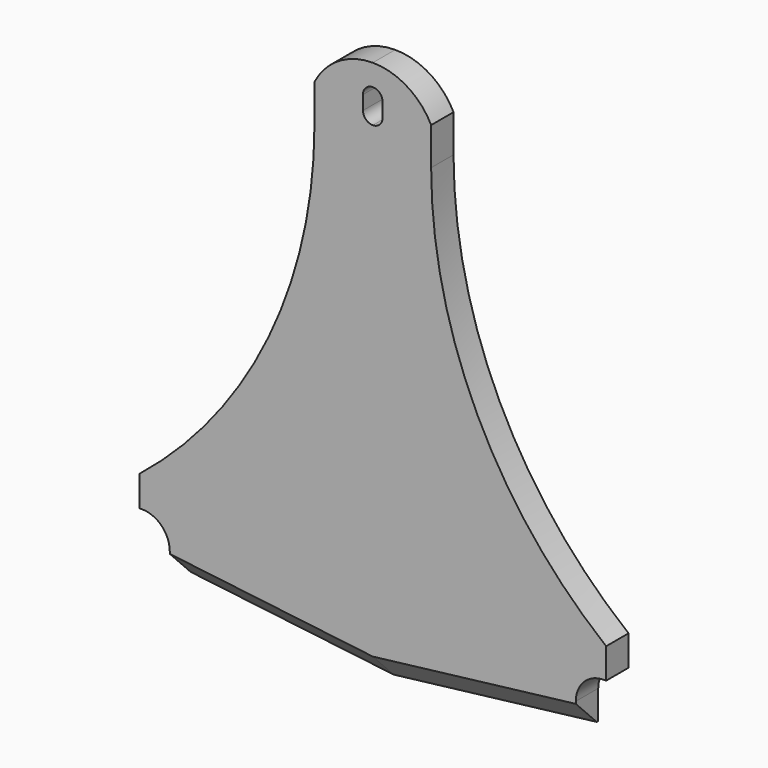
from build123d import *

# Parameters (mm, degrees)
F1_DEPTH    = 6
F2_R        = 6
F3_SIZE2    = 5.6
F3_SIZE     = 5.64
F4_T1_DEPTH = 6


# Not quite as in the source:
# - a fillet or chamfer that OpenCascade refuses, or shapes differently, is made with other operations: its cross-section is extruded or revolved along the edge and cut away or added


with BuildPart() as f1:
    # F0 (on Front) → F1 (new body)
    with BuildSketch(Plane.XZ):
        with BuildLine():
            Line((-43.5, -10.06), (0, -15.282))
            Line((0, -15.282), (0, 74.41))
            ThreePointArc((0, 74.41), (-7.3393922947, 76.4880320104), (-12.5, 82.1052398935))
            Line((-12.5, 82.1052398935), (-12.5, 8.61))
            Line((-12.5, 8.61), (-50, 8.61))
            Line((-50, 8.61), (-50, 2.11))
            Line((-50, 2.11), (-43.5, 2.11))
            Line((-43.5, 2.11), (-43.5, -10.06))
        make_face()
        with BuildLine():
            ThreePointArc((-12.5, 82.1052398935), (-7.3393922947, 76.4880320104), (0, 74.41))
            Line((0, 74.41), (0, 90.615))
            ThreePointArc((0, 90.615), (-1.4849242405, 91.2300757595), (-2.1, 92.715))
            Line((-2.1, 92.715), (-2.1, 95.715))
            ThreePointArc((-2.1, 95.715), (-1.4849242405, 97.1999242405), (0, 97.815))
            Line((0, 97.815), (0, 102.41))
            ThreePointArc((0, 102.41), (-7.3393922947, 100.3319679896), (-12.5, 94.7147601065))
            Line((-12.5, 94.7147601065), (-12.5, 82.1052398935))
        make_face()
    extrude(amount=-F1_DEPTH)

    # F2
    f2_edges = [f1.edges().sort_by_distance(p)[0] for p in [
        (-43.5, 3, 2.11),
    ]]
    fillet(f2_edges, radius=F2_R)

    # F3
    f3_edges = [f1.edges().sort_by_distance(p)[0] for p in [
        (-21.75, 0, -12.671),
    ]]
    f3_side = f1.faces().sort_by_distance((-42.221274, 0, -6.975))[0]
    chamfer(f3_edges, length=F3_SIZE, length2=F3_SIZE2, reference=f3_side)

    # F4: fillet of radius 100 on 1 edges, made by hand

    # F4_s2 → F4_t1 (join)
    with BuildSketch(Plane.XZ.offset(-6)):
        with BuildLine():
            ThreePointArc((-50, 8.61), (-22.3612181134, 43.3712047908), (-12.5, 86.67247498))
            Line((-12.5, 86.67247498), (-12.5, 8.61))
            Line((-12.5, 8.61), (-50, 8.61))
        make_face()
    extrude(amount=F4_T1_DEPTH)

    # F5: F1 across plane


with BuildPart() as f1_1:
    add(f1.part)
    add(f1.part.mirror(Plane.YZ))


solid = f1_1.part
